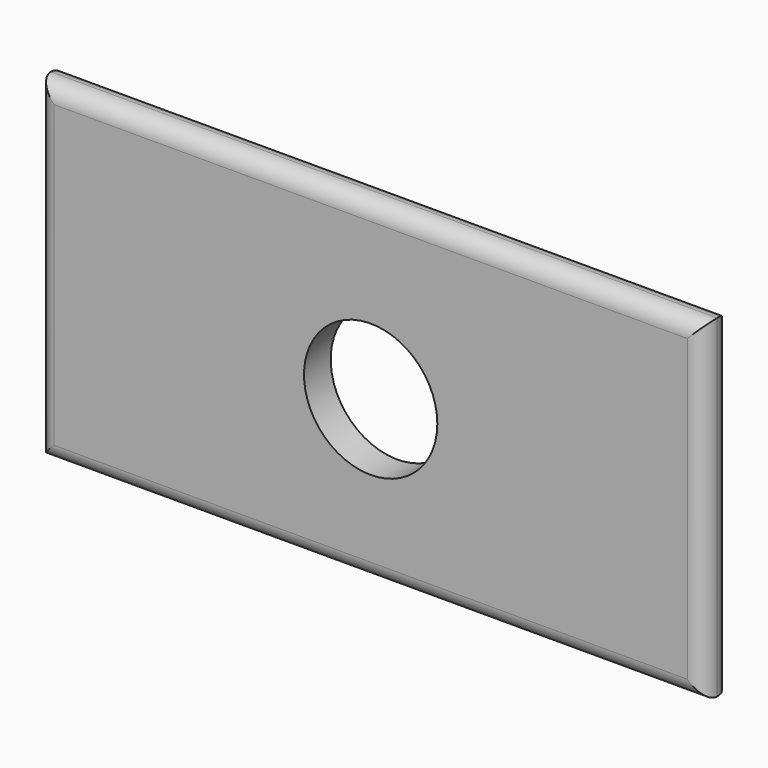
from build123d import *

# Parameters (mm, degrees)
F0_W     = 200
F0_H     = 100
F1_DEPTH = 10
F2_R     = 20
F3_DEPTH = 10.001
F4_R     = 4.99999


# Not quite as in the source:
# - a fillet or chamfer is up to 0.001 mm smaller than in the source, because OpenCascade refuses the exact size


with BuildPart() as f1:
    # F0 (on Front) → F1 (new body)
    with BuildSketch(Plane.XZ):
        Rectangle(F0_W, F0_H)
    extrude(amount=F1_DEPTH)

    # F2 (on face) → F3 (cut, through all)
    with BuildSketch(Plane.XZ.offset(10)):
        with Locations((0, -1.9458576571)):
            Circle(F2_R)
    extrude(amount=-F3_DEPTH, mode=Mode.SUBTRACT)

    # F4 (radius 5 in the source; OpenCascade refuses exactly that, so slightly less here)
    f4_edges = [f1.edges().sort_by_distance(p)[0] for p in [
        (0, -10, 50),
        (0, 0, 50),
        (100, 0, 0),
        (100, -10, 0),
        (0, -10, -50),
        (-100, -10, 0),
    ]]
    fillet(f4_edges, radius=F4_R)


solid = f1.part
